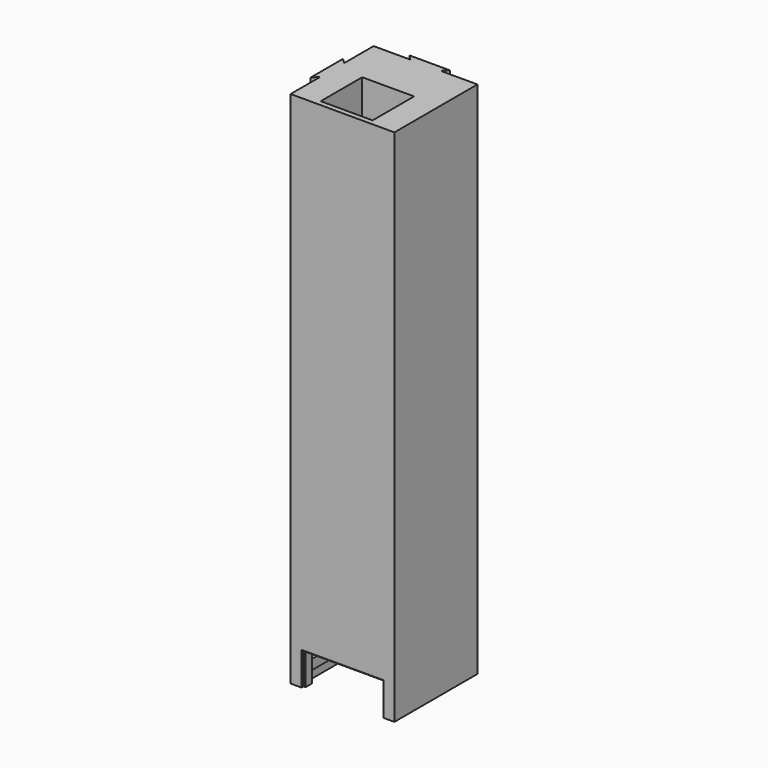
from build123d import *

# Parameters (mm, degrees)
F0_W     = 12.7
F0_H     = 12.7
F1_DEPTH = 127
F2_W     = 12.7
F2_H     = 12.7
F3_DEPTH = 7.62
F5_DEPTH = 0.635
F6_W     = 20.32
F6_H     = 2.413
F7_DEPTH = 1.016


# Not quite as in the source:
# - a feature names something its author has since deleted; it is built from what else it names


with BuildPart() as f1:
    # F0 (on Top) → F1 (new body)
    with BuildSketch(Plane.XY):
        Polygon((-13.97, -4.953), (-12.7, -3.683), (-12.7, 3.683), (-13.97, 4.953), align=None)
        Polygon((-3.683, 12.7), (3.683, 12.7), (4.953, 13.97), (-4.953, 13.97), align=None)
        Polygon((12.7, -12.7), (12.7, 12.7), (3.683, 12.7), (-3.683, 12.7), (-12.7, 12.7), (-12.7, 3.683), (-12.7, -3.683), (-12.7, -12.7), align=None)
        with Locations((0, -5.08)):
            Rectangle(F0_W, F0_H, mode=Mode.SUBTRACT)
    extrude(amount=F1_DEPTH)

    # F2 (on face) → F3 (cut)
    with BuildSketch(Plane(origin=(0, 0, 0), x_dir=(1, 0, 0), z_dir=(0, 0, -1))):
        Polygon((9.525, 12.7), (-9.525, 12.7), (-9.525, 10.16), (-10.795, 10.16), (-10.795, -10.16), (10.795, -10.16), (10.795, 10.16), (9.525, 10.16), align=None)
        with Locations((0, 5.08)):
            Rectangle(F2_W, F2_H, mode=Mode.SUBTRACT)
    extrude(amount=-F3_DEPTH, mode=Mode.SUBTRACT)

    # F4 (on face) → F5 (cut)
    with BuildSketch(Plane.XZ.offset(12.7)):
        Polygon((10.033, 8.128), (-10.033, 8.128), (-10.033, 0), (-9.525, 0), (-9.525, 7.62), (9.525, 7.62), (9.525, 0), (10.033, 0), align=None)
    extrude(amount=-F5_DEPTH, mode=Mode.SUBTRACT)



with BuildPart() as f7:
    # F6 (on face) → F7 (new body)
    with BuildSketch(Plane.YZ.offset(-10.795)):
        with Locations((0, 3.8735)):
            Rectangle(F6_W, F6_H)
    extrude(amount=F7_DEPTH)


with BuildPart() as f1_1:
    add(f1.part)

    add(f7.part)  # F8 merges F7
    # F8: F7 across plane
    add(f7.part.mirror(Plane.YZ))


with BuildPart() as f9_1:
    # F9: copy of F1
    add(f1_1.part)


solid = f1_1.part
